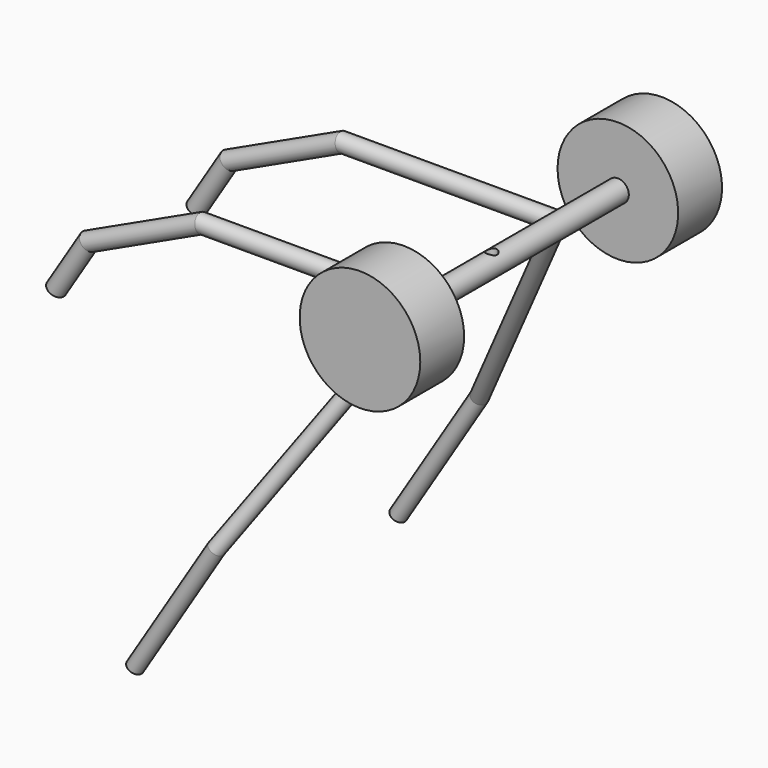
from build123d import *

# Parameters (mm, degrees)
F2_R           = 4
F9_R           = 3.5
F5_R           = 5
F12_DEPTH      = 50
F12_DEPTH_BACK = 72
F13_R          = 2.5
F14_DEPTH      = 166.5263197276
F14_DEPTH_BACK = 5.0010001
F15_R          = 27.5
F16_DEPTH      = 25
F17_R          = 27.5
F18_DEPTH      = 25


with BuildPart() as f3:
    # F3: sweep along a path in F1
    with BuildLine(Plane.XZ) as f3_path:
        Line((0, 0), (-100, 0))
        Line((-100, 0), (-151.6595438611, -24.0892409192))
        Line((-151.6595438611, -24.0892409192), (-166.4617190554, -47.8567735955))
    # F2 (on Right) → F3 (sweep)
    with BuildSketch(Plane.YZ):
        with Locations((-4, 0)):
            Circle(F2_R)
        with Locations((-84, 0)):
            Circle(F2_R)
    sweep(path=f3_path.line, transition=Transition.RIGHT)

    # F10: sweep along a path in F8
    with BuildLine(Plane(origin=(0, 0, 0), x_dir=(0, -1, 0), z_dir=(-0.8488404527, 0, 0.5286491141))) as f10_path:
        Line((44, 0), (80.5, 0))
        Line((80.5, 0), (119, -124))
        Line((119, -124), (119, -194))
    # F9 (on mid) → F10 (sweep)
    with BuildSketch(Plane.XZ.offset(44)):
        Circle(F9_R)
    sweep(path=f10_path.line, transition=Transition.RIGHT)

    # F11: F3 across plane


with BuildPart() as f3_1:
    add(f3.part)
    add(f3.part.mirror(Plane.XZ.offset(44)))

    # F5 (on mid) → F12 (join, two sides)
    with BuildSketch(Plane.XZ.offset(44)) as f12_sk:
        Circle(F5_R)
    extrude(amount=F12_DEPTH)
    extrude(f12_sk.sketch, amount=-F12_DEPTH_BACK)

    # F13 (on Top) → F14 (cut, two sides)
    with BuildSketch(Plane.XY) as f14_sk:
        with Locations((0, -44)):
            Circle(F13_R)
    extrude(amount=-F14_DEPTH, mode=Mode.SUBTRACT)
    extrude(f14_sk.sketch, amount=F14_DEPTH_BACK, mode=Mode.SUBTRACT)

    # F15 (on face) → F16 (join)
    with BuildSketch(Plane.XZ.offset(94)):
        Circle(F15_R)
    extrude(amount=F16_DEPTH)

    # F17 (on face) → F18 (join)
    with BuildSketch(Plane(origin=(0, 28, 0), x_dir=(-1, 0, 0), z_dir=(0, 1, 0))):
        Circle(F17_R)
    extrude(amount=F18_DEPTH)


solid = f3_1.part
